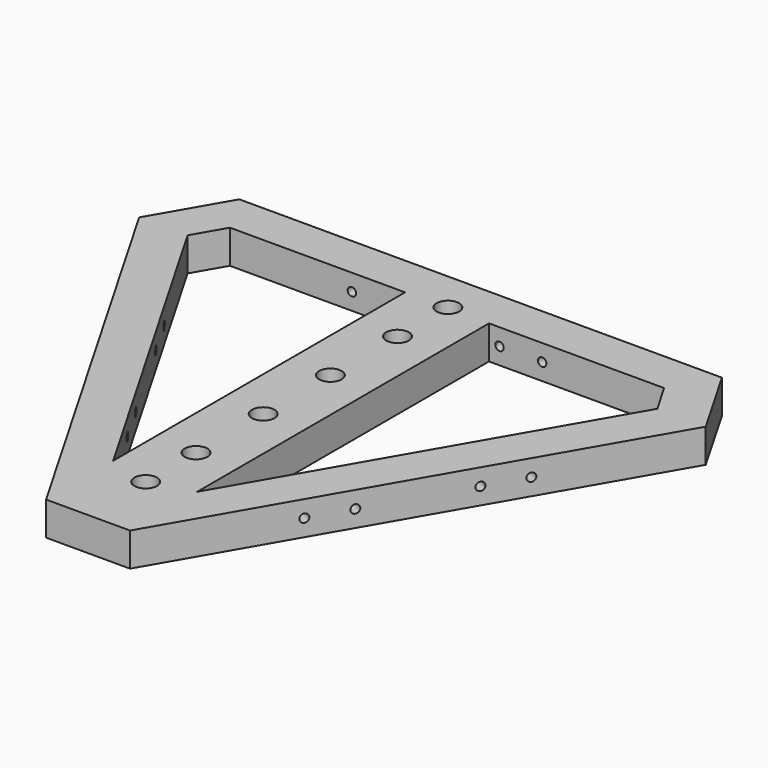
from build123d import *

# Parameters (mm, degrees)
F0_R            = 2.7
F1_DEPTH        = 8
F2_R            = 1
F3_DEPTH        = 11
F3_COPIES_COUNT = 3


# Not quite as in the source:
# - a pattern or mirror of a feature is missing from the dataset's text; its kind, count and spacing are read off the source's solid


with BuildPart() as f1:
    # F0 (on Top) → F1 (new body)
    with BuildSketch(Plane.XY):
        Polygon((57.5, 58.4567147554), (-57.5, 58.4567147554), (-67.5, 41.1362066798), (-10, -58.4567147554), (10, -58.4567147554), (67.5, 41.1362066798), align=None)
        with Locations((0, -41.2879311067)):
            Circle(F0_R, mode=Mode.SUBTRACT)
        with Locations((0, -26.2879311067)):
            Circle(F0_R, mode=Mode.SUBTRACT)
        with Locations((0, -6.2879311067)):
            Circle(F0_R, mode=Mode.SUBTRACT)
        Polygon((-10, 48.4567147554), (-10, -38.4567147554), (-55.9529946162, 41.1362066798), (-51.7264973081, 48.4567147554), align=None, mode=Mode.SUBTRACT)
        with Locations((0, 13.7120688933)):
            Circle(F0_R, mode=Mode.SUBTRACT)
        Polygon((51.7264973081, 48.4567147554), (55.9529946162, 41.1362066798), (10, -38.4567147554), (10, 48.4567147554), align=None, mode=Mode.SUBTRACT)
        with Locations((0, 33.7120688933)):
            Circle(F0_R, mode=Mode.SUBTRACT)
        with Locations((0, 48.7120688933)):
            Circle(F0_R, mode=Mode.SUBTRACT)
    extrude(amount=F1_DEPTH)

    # F2 (on face) → F3 (cut)
    with BuildSketch(Plane(origin=(32.8125, -18.9443057078, 0), x_dir=(0.5, 0.8660254038, 0), z_dir=(0.8660254038, -0.5, 0))):
        with Locations((-10.795, 4)):
            Circle(F2_R)
        with Locations((-0.625, 4)):
            Circle(F2_R)
        with Locations((34.545, 4)):
            Circle(F2_R)
        with Locations((24.375, 4)):
            Circle(F2_R)
    f3 = extrude(amount=-F3_DEPTH, mode=Mode.SUBTRACT)

    # F3_copies: F3 ×3 about axis
    f3_copies_axis = Axis((0, 13.712069, 0), (0, 0, 1))
    for i in range(1, F3_COPIES_COUNT):
        add(f3.rotate(f3_copies_axis, i * 360 / F3_COPIES_COUNT), mode=Mode.SUBTRACT)


solid = f1.part
